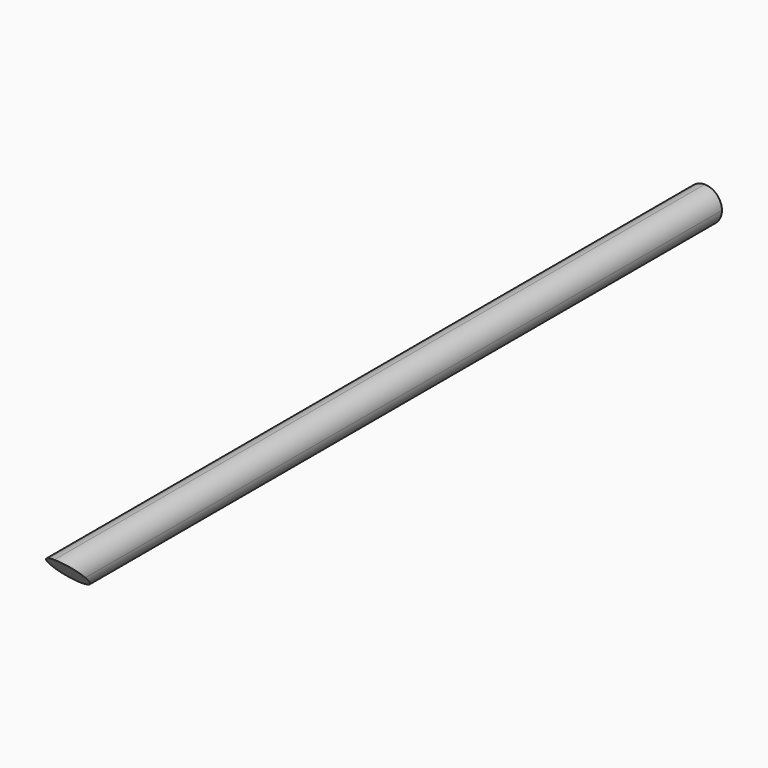
from build123d import *

# Parameters (mm, degrees)
F0_W     = 42
F0_H     = 42
F1_DEPTH = 992
F3_DEPTH = 100
F4_R     = 20.99999


# Not quite as in the source:
# - a fillet or chamfer is up to 0.001 mm smaller than in the source, because OpenCascade refuses the exact size


with BuildPart() as f1:
    # F0 (on Front) → F1 (new body)
    with BuildSketch(Plane.XZ):
        Rectangle(F0_W, F0_H)
    extrude(amount=F1_DEPTH)

    # F2 (on face) → F3 (cut)
    with BuildSketch(Plane.YZ.offset(21)):
        Polygon((-950, -21), (-992, 21), (-992, -21), align=None)
    extrude(amount=-F3_DEPTH, mode=Mode.SUBTRACT)

    # F4 (radius 21 in the source; OpenCascade refuses exactly that, so slightly less here)
    f4_edges = [f1.edges().sort_by_distance(p)[0] for p in [
        (-21, -496, 21),
        (-21, -475, -21),
        (21, -496, 21),
        (21, -475, -21),
    ]]
    fillet(f4_edges, radius=F4_R)


solid = f1.part
